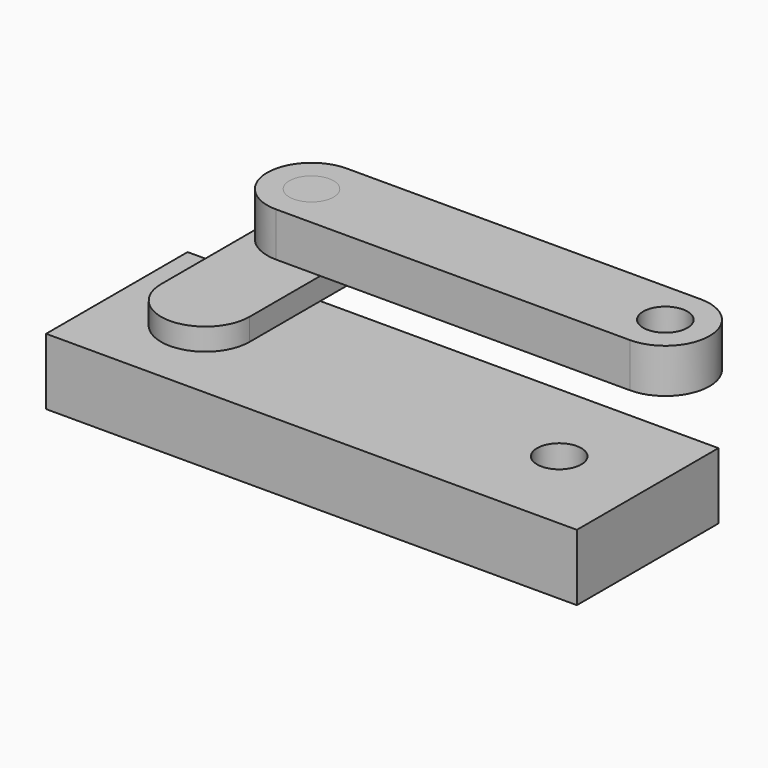
from build123d import *

# Parameters (mm, degrees)
F0_W          = 120
F0_H          = 40
F0_R          = 5
F1_DEPTH      = 15
F2_R          = 5
F3_DEPTH      = 5
F4_DEPTH      = 15
F5_DEPTH      = 5
F5_DEPTH_BACK = 10
F6_R          = 5
F7_DEPTH      = 10


with BuildPart() as f1:
    # F0 (on Top) → F1 (new body)
    with BuildSketch(Plane.XY):
        with Locations((60, 20)):
            Rectangle(F0_W, F0_H)
        with Locations((20, 20)):
            Circle(F0_R, mode=Mode.SUBTRACT)
        with Locations((100, 20)):
            Circle(F0_R, mode=Mode.SUBTRACT)
    extrude(amount=F1_DEPTH)


with BuildPart() as f3:
    # F2 (on face) → F3 (new body)
    with BuildSketch(Plane.XY.offset(15)):
        with BuildLine():
            Line((30, 20), (30, 50))
            ThreePointArc((30, 50), (20, 60), (10, 50))
            Line((10, 50), (10, 20))
            ThreePointArc((10, 20), (20, 10), (30, 20))
        make_face()
        with Locations((20, 20)):
            Circle(F2_R, mode=Mode.SUBTRACT)
        with Locations((20, 50)):
            Circle(F2_R, mode=Mode.SUBTRACT)
    extrude(amount=F3_DEPTH)

    # F2 (on face) → F4 (join)
    with BuildSketch(Plane.XY.offset(15)):
        with Locations((20, 50)):
            Circle(F2_R)
    extrude(amount=F4_DEPTH)

    # F2 (on face) → F5 (join, two sides)
    with BuildSketch(Plane.XY.offset(15)) as f5_sk:
        with Locations((20, 20)):
            Circle(F2_R)
    extrude(amount=F5_DEPTH)
    extrude(f5_sk.sketch, amount=-F5_DEPTH_BACK)


with BuildPart() as f7:
    # F6 (on face) → F7 (new body)
    with BuildSketch(Plane.XY.offset(20)):
        with BuildLine():
            Line((100, 60), (20, 60))
            ThreePointArc((20, 60), (27.0710678119, 57.0710678119), (30, 50))
            Line((30, 50), (30, 40))
            Line((30, 40), (100, 40))
            ThreePointArc((100, 40), (110, 50), (100, 60))
        make_face()
        with Locations((100, 50)):
            Circle(F6_R, mode=Mode.SUBTRACT)
        with BuildLine():
            ThreePointArc((30, 50), (27.0710678119, 57.0710678119), (20, 60))
            ThreePointArc((20, 60), (12.9289321881, 57.0710678119), (10, 50))
            ThreePointArc((10, 50), (12.9289321881, 42.9289321881), (20, 40))
            Line((20, 40), (30, 40))
            Line((30, 40), (30, 50))
        make_face()
        with Locations((20, 50)):
            Circle(F6_R, mode=Mode.SUBTRACT)
    extrude(amount=F7_DEPTH)


solid = Compound([f1.part, f3.part, f7.part])
